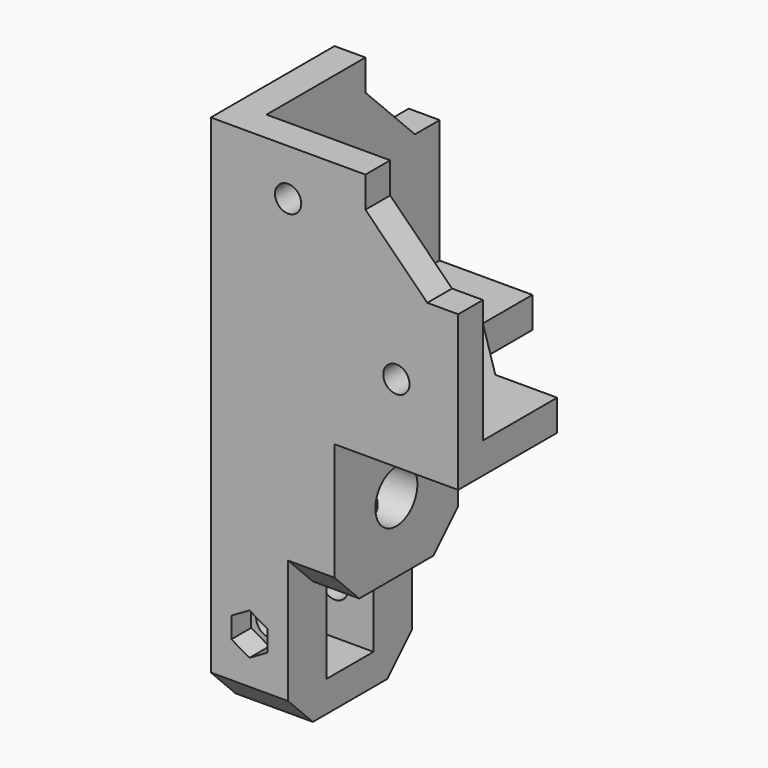
from build123d import *

# Parameters (mm, degrees)
F0_R         = 2.125
F1_DEPTH     = 5
F3_DEPTH     = 20
F5_DEPTH     = 15
F6_SIZE      = 10
F7_R         = 2.125
F8_DEPTH     = 5
F9_R         = 2.125
F10_DEPTH    = 5
F11_W        = 40
F11_H        = 20
F11_R        = 2.125
F12_DEPTH    = 24
F14_DEPTH    = 25
F15_R        = 4.25
F16_DEPTH    = 20
F17_R        = 3.5
F18_DEPTH    = 25
F19_W        = 20
F19_H        = 24
F20_DEPTH    = 5
F22_DEPTH    = 12.5
F23_T4_DEPTH = 20
F23_S5_R     = 2.125
F23_T6_DEPTH = 12
F23_T7_DEPTH = 38.2168298797
F23_T9_DEPTH = 20.3584149398
F24_R        = 3.5
F25_DEPTH    = 44.001
F26_R        = 4.25
F26_R_2      = 1.6
F27_DEPTH    = 5
F28_R        = 2.125
F29_DEPTH    = 40.001
F31_DEPTH    = 4
F32_R        = 3.5
F33_DEPTH    = 4


# Not quite as in the source:
# - a fillet or chamfer that OpenCascade refuses, or shapes differently, is made with other operations: its cross-section is extruded or revolved along the edge and cut away or added


with BuildPart() as f1:
    # F0 (on Top) → F1 (new body)
    with BuildSketch(Plane.XY):
        Polygon((0, 20), (0, 40), (-20, 40), (-20, 0), (20, 0), (20, 20), align=None)
        with Locations((-7.5, 12.5)):
            Circle(F0_R, mode=Mode.SUBTRACT)
        with Locations((10, 12.5)):
            Circle(F0_R, mode=Mode.SUBTRACT)
        with Locations((-7.5, 30)):
            Circle(F0_R, mode=Mode.SUBTRACT)
    extrude(amount=F1_DEPTH)

    # F2 (on face) → F3 (join)
    with BuildSketch(Plane.XY.offset(5)):
        Polygon((-15, 40), (-20, 40), (-20, 0), (20, 0), (20, 5), (-15, 5), align=None)
    extrude(amount=F3_DEPTH)

    # F4 (on face) → F5 (join)
    with BuildSketch(Plane.XY.offset(25)):
        Polygon((-15, 5), (-15, 25), (-20, 25), (-20, 0), (5, 0), (5, 5), align=None)
    extrude(amount=F5_DEPTH)

    # F6
    f6_edges = [f1.edges().sort_by_distance(p)[0] for p in [
        (0, 20, 2.5),
        (-17.5, 25, 25),
        (5, 2.5, 25),
    ]]
    chamfer(f6_edges, length=F6_SIZE)

    # F7 (on face) → F8 (cut)
    with BuildSketch(Plane.XZ):
        with Locations((-7.5, 32.5)):
            Circle(F7_R)
        with Locations((10, 12.5)):
            Circle(F7_R)
    extrude(amount=-F8_DEPTH, mode=Mode.SUBTRACT)

    # F9 (on face) → F10 (cut)
    with BuildSketch(Plane(origin=(-20, 0, 0), x_dir=(0, -1, 0), z_dir=(-1, 0, 0))):
        with Locations((-12.5, 32.5)):
            Circle(F9_R)
        with Locations((-30, 12.5)):
            Circle(F9_R)
    extrude(amount=-F10_DEPTH, mode=Mode.SUBTRACT)

    # F11 (on face) → F12 (join)
    with BuildSketch(Plane(origin=(0, 0, 0), x_dir=(1, 0, 0), z_dir=(0, 0, -1))):
        with Locations((0, -10)):
            Rectangle(F11_W, F11_H)
        with Locations((-7.5, -12.5)):
            Circle(F11_R, mode=Mode.SUBTRACT)
        with Locations((10, -12.5)):
            Circle(F11_R, mode=Mode.SUBTRACT)
    extrude(amount=F12_DEPTH)

    # F13 (on face) → F14 (cut)
    with BuildSketch(Plane(origin=(0, 20, 0), x_dir=(-1, 0, 0), z_dir=(0, 1, 0))):
        Polygon((0, -24), (0, -11.5), (0, 0), (-20, 0), (-20, -24), align=None)
    extrude(amount=-F14_DEPTH, mode=Mode.SUBTRACT)

    # F15 (on face) → F16 (cut)
    with BuildSketch(Plane.YZ):
        with Locations((12.5, -12.5)):
            Circle(F15_R)
    extrude(amount=-F16_DEPTH, mode=Mode.SUBTRACT)

    # F17 (on face) → F18 (cut)
    with BuildSketch(Plane(origin=(0, 0, -24), x_dir=(1, 0, 0), z_dir=(0, 0, -1))):
        with Locations((-7.5, -12.5)):
            Circle(F17_R)
    extrude(amount=-F18_DEPTH, mode=Mode.SUBTRACT)

    # F19 (on face) → F20 (join)
    with BuildSketch(Plane(origin=(0, 20, 0), x_dir=(-1, 0, 0), z_dir=(0, 1, 0))):
        with Locations((10, -12)):
            Rectangle(F19_W, F19_H)
    extrude(amount=F20_DEPTH)

    # F21 (on face) → F22 (join)
    with BuildSketch(Plane(origin=(-20, 0, 0), x_dir=(0, -1, 0), z_dir=(-1, 0, 0))):
        Polygon((-17.25, -24), (-25, -24), (-25, -44), (0, -44), (0, -24), (-7.75, -24), (-7.75, -39), (-17.25, -39), align=None)
    extrude(amount=-F22_DEPTH)

    # F23: chamfer of 5 on 5 edges, made by hand


with BuildPart() as f23_tool2:
    # F23_s3 → F23_t4 (new body)
    with BuildSketch(Plane.YZ.offset(-20)):
        Polygon((25, -5), (30, 0), (25, 0), align=None)
    extrude(amount=F23_T4_DEPTH)

    # F23_s5 → F23_t6 (cut, symmetric)
    with BuildSketch(Plane.XY.offset(-2.5)):
        with Locations((-7.5, 30)):
            Circle(F23_S5_R)
    extrude(amount=F23_T6_DEPTH, both=True, mode=Mode.SUBTRACT)


with BuildPart() as f1_1:
    add(f1.part)

    # F23_t1: union F23_tool2
    add(f23_tool2.part)

    # F23_s8 → F23_t7 (cut)
    with BuildSketch(Plane.YZ.offset(-32.8584149398)):
        Polygon((25, -39), (20, -44), (25, -44), align=None)
        Polygon((0, -39), (5, -44), (0, -44), align=None)
    extrude(amount=F23_T7_DEPTH, mode=Mode.SUBTRACT)

    # F23_s10 → F23_t9 (cut)
    with BuildSketch(Plane.YZ.offset(-7.5)):
        Polygon((5, -24), (0, -19), (0, -24), align=None)
        Polygon((25, -19), (20, -24), (25, -24), align=None)
    extrude(amount=F23_T9_DEPTH, mode=Mode.SUBTRACT)

    # F24 (on face) → F25 (cut, through all)
    with BuildSketch(Plane(origin=(0, 0, 0), x_dir=(1, 0, 0), z_dir=(0, 0, -1))):
        with Locations((-7.5, -30)):
            Circle(F24_R)
    extrude(amount=F25_DEPTH, mode=Mode.SUBTRACT)

    # F26 (on face) → F27 (join)
    with BuildSketch(Plane(origin=(-20, 0, 0), x_dir=(0, -1, 0), z_dir=(-1, 0, 0))):
        with Locations((-12.5, -12.5)):
            Circle(F26_R)
        with Locations((-12.5, -12.5)):
            Circle(F26_R_2, mode=Mode.SUBTRACT)
    extrude(amount=-F27_DEPTH)

    # F28 (on face) → F29 (cut, through all)
    with BuildSketch(Plane.XZ):
        with Locations((-13.75, -31.5)):
            Circle(F28_R)
    extrude(amount=-F29_DEPTH, mode=Mode.SUBTRACT)

    # F30 (on face) → F31 (cut)
    with BuildSketch(Plane.XZ):
        Polygon((-10.825, -33.1887495374), (-10.825, -29.8112504626), (-13.75, -28.1225009252), (-16.675, -29.8112504626), (-16.675, -33.1887495374), (-13.75, -34.8774990748), align=None)
    extrude(amount=-F31_DEPTH, mode=Mode.SUBTRACT)

    # F32 (on face) → F33 (cut)
    with BuildSketch(Plane(origin=(0, 25, 0), x_dir=(-1, 0, 0), z_dir=(0, 1, 0))):
        with Locations((13.75, -31.5)):
            Circle(F32_R)
    extrude(amount=-F33_DEPTH, mode=Mode.SUBTRACT)


solid = f1_1.part
